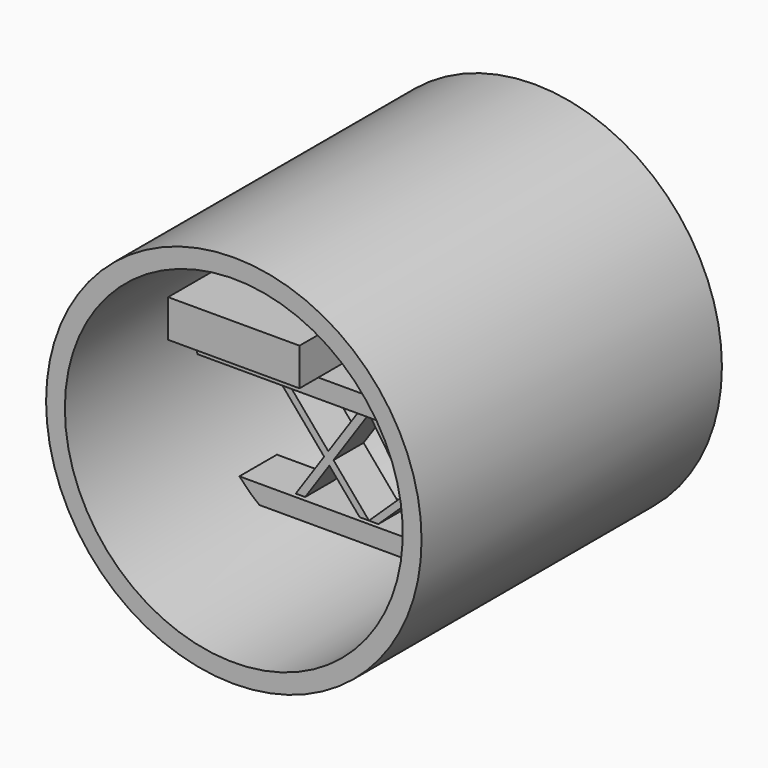
from build123d import *

# Parameters (mm, degrees)
F0_R     = 100
F1_DEPTH = 100
F2_R     = 90
F3_DEPTH = 200
F5_DEPTH = 100
F4_W     = 4.9999998882
F4_H     = 50
F4_W_2   = 5
F6_DEPTH = 5
F7_DEPTH = 12.5
F8_DEPTH = 10


# Not quite as in the source:
# - a feature names something its author has since deleted; it is built from what else it names


with BuildPart() as f1:
    # F0 (on Front) → F1 (new body, symmetric)
    with BuildSketch(Plane.XZ):
        Circle(F0_R)
    extrude(amount=F1_DEPTH, both=True)

    # F2 (on face) → F3 (cut)
    with BuildSketch(Plane(origin=(0, 100, 0), x_dir=(-1, 0, 0), z_dir=(0, 1, 0))):
        Circle(F2_R)
    extrude(amount=-F3_DEPTH, mode=Mode.SUBTRACT)


with BuildPart() as f5:
    # F4 (on Front) → F5 (new body, symmetric)
    with BuildSketch(Plane.XZ):
        Polygon((-4.9999998882, 50), (0, 50), (5, 50), (35, 50), (35, 70), (-35, 70), (-35, 50), align=None)
    extrude(amount=F5_DEPTH, both=True)

    # F4 (on Front) → F6 (join, symmetric)
    with BuildSketch(Plane.XZ):
        with Locations((-2.4999999441, 25)):
            Rectangle(F4_W, F4_H)
        with Locations((2.5, 25)):
            Rectangle(F4_W_2, F4_H)
    extrude(amount=F6_DEPTH, both=True)


with BuildPart() as f7:
    # F4 (on Front) → F7 (new body, symmetric)
    with BuildSketch(Plane.XZ):
        Polygon((5, 0), (0, 0), (-4.9999998882, 0), (-90, 0), (-90, -10), (-47.5, -10), (-42.5, -10), (-40.6034433022, -10), (-5, -10), (0, -10), (5, -10), (52.3540072756, -10), (52.5, -9.8605715856), (57.5, -9.8458949104), (57.3386868395, -10), (90, -10), (90, 0), (45, 0), align=None)
    extrude(amount=F7_DEPTH, both=True)


with BuildPart() as f7b:
    # F4 (on Front) → F7, piece 2 (new body, symmetric)
    with BuildSketch(Plane.XZ):
        Polygon((-34, -60), (-39, -60), (-64.5170719501, -60), (-68, -60), (-68, -70), (0, -70), (68, -70), (68, -60), (39, -60), (34, -60), (5, -60), (0, -60), (-5, -60), align=None)
    extrude(amount=F7_DEPTH, both=True)


with BuildPart() as f8:
    # F4 (on Front) → F8 (new body, symmetric)
    with BuildSketch(Plane.XZ):
        Polygon((-42.5, -10), (-47.5, -10), (-23.8888888889, -37.7777777778), (-21.6666666667, -34.5098039216), align=None)
        Polygon((-21.1111111111, -41.045751634), (-23.8888888889, -37.7777777778), (-39, -60), (-34, -60), align=None)
        Polygon((-21.6666666667, -34.5098039216), (-23.8888888889, -37.7777777778), (-21.1111111111, -41.045751634), (-18.8888888889, -37.7777777778), align=None)
        Polygon((-5, -10), (-21.6666666667, -34.5098039216), (-18.8888888889, -37.7777777778), (0, -10), align=None)
        Polygon((-18.8888888889, -37.7777777778), (-21.1111111111, -41.045751634), (-5, -60), (0, -60), align=None)
    extrude(amount=F8_DEPTH, both=True)


with BuildPart() as f8b:
    # F4 (on Front) → F8, piece 2 (new body, symmetric)
    with BuildSketch(Plane.XZ):
        Polygon((5, -60), (22.579858739, -43.2056746161), (20.6132442897, -40.3135945437), (0, -60), align=None)
        Polygon((22.579858739, -43.2056746161), (25.6108688664, -40.3101012741), (23.6446037441, -37.4185349178), (20.6132442897, -40.3135945437), align=None)
        Polygon((39, -60), (25.6108688664, -40.3101012741), (22.579858739, -43.2056746161), (34, -60), align=None)
        Polygon((52.3540072756, -10), (57.3386868395, -10), (57.5, -9.8458949104), (52.5, -9.8605715856), align=None)
        Polygon((20.6132442897, -40.3135945437), (23.6446037441, -37.4185349178), (5, -10), (0, -10), align=None)
        Polygon((25.6108688664, -40.3101012741), (57.3386868395, -10), (52.3540072756, -10), (23.6446037441, -37.4185349178), align=None)
    extrude(amount=F8_DEPTH, both=True)


solid = Compound([f1.part, f5.part, f7.part, f7b.part, f8.part, f8b.part])
